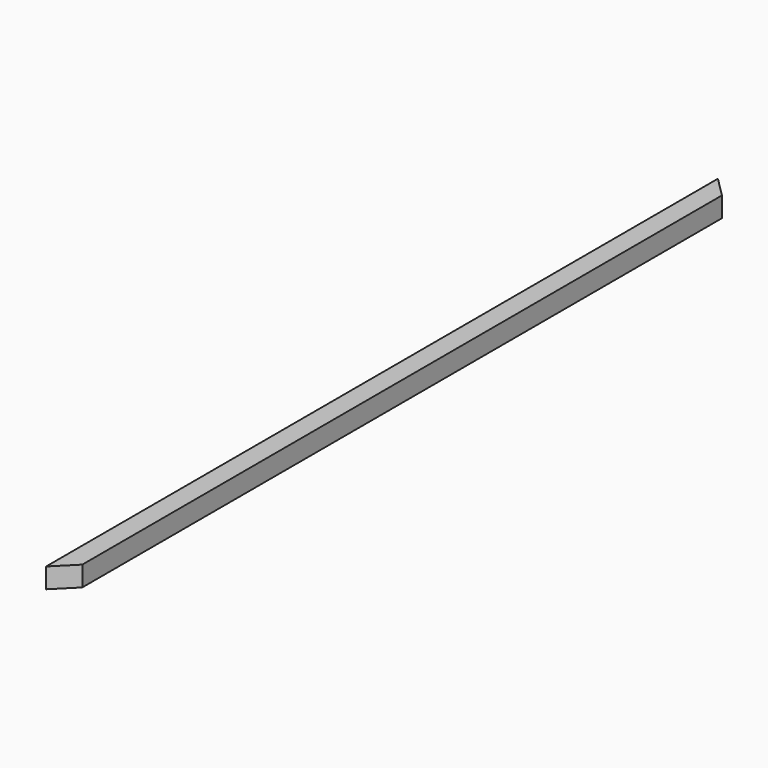
from build123d import *

# Parameters (mm, degrees)
F0_W     = 20
F0_H     = 20
F1_DEPTH = 417.793
F2_SIZE2 = 19.99999
F2_SIZE  = 19.99999
F3_SIZE  = 19.99999
F4_R     = 3
F5_DEPTH = 4
F6_R     = 3
F7_DEPTH = 4


# Not quite as in the source:
# - a fillet or chamfer is up to 0.001 mm smaller than in the source, because OpenCascade refuses the exact size


with BuildPart() as f1:
    # F0 (on Front) → F1 (new body, symmetric)
    with BuildSketch(Plane.XZ):
        with Locations((10, 10)):
            Rectangle(F0_W, F0_H)
    extrude(amount=F1_DEPTH, both=True)

    # F2 (size 20 and 20 in the source; OpenCascade refuses exactly that, so slightly less here)
    f2_edges = [f1.edges().sort_by_distance(p)[0] for p in [
        (20, -417.793, 10),
    ]]
    chamfer(f2_edges, length=F2_SIZE, length2=F2_SIZE2)

    # F3 (size 20 in the source; OpenCascade refuses exactly that, so slightly less here)
    f3_edges = [f1.edges().sort_by_distance(p)[0] for p in [
        (20, 417.793, 10),
    ]]
    chamfer(f3_edges, length=F3_SIZE)

    # F4 (on face) → F5 (cut)
    with BuildSketch(Plane(origin=(0, 0, 0), x_dir=(0, -1, 0), z_dir=(-1, 0, 0))):
        with Locations((-407.793, 10)):
            Circle(F4_R)
    extrude(amount=-F5_DEPTH, mode=Mode.SUBTRACT)

    # F6 (on face) → F7 (cut)
    with BuildSketch(Plane(origin=(0, 0, 0), x_dir=(0, -1, 0), z_dir=(-1, 0, 0))):
        with Locations((407.793, 10)):
            Circle(F6_R)
    extrude(amount=-F7_DEPTH, mode=Mode.SUBTRACT)


solid = f1.part
